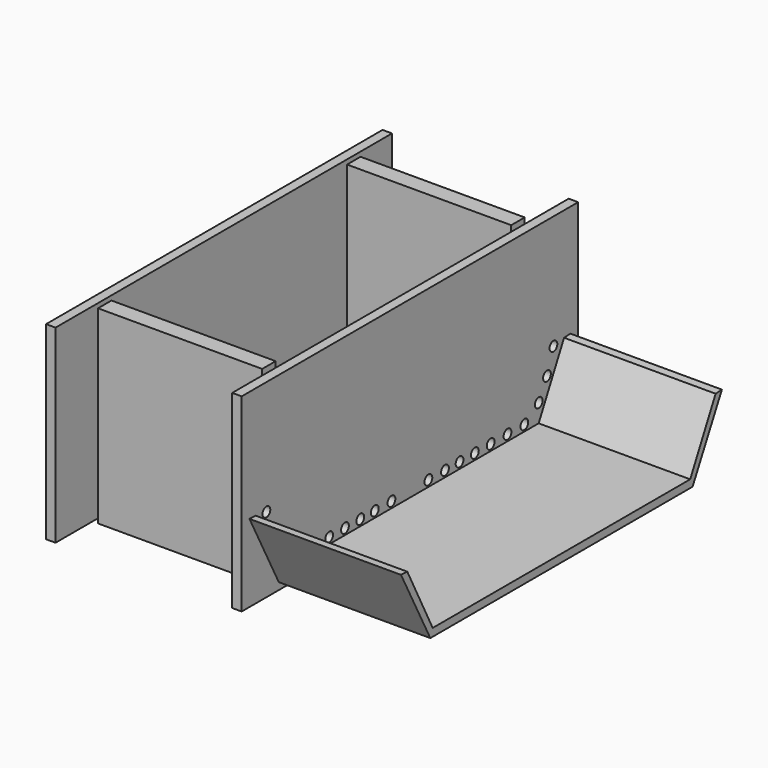
from build123d import *

# Parameters (mm, degrees)
F0_W     = 21.6278625545
F0_H     = 77.5424886208
F1_DEPTH = 10
F0_W_2   = 43.3333408518
F0_H_2   = 4.4457448224
F2_DEPTH = 50
F3_R     = 1.2843906964
F4_DEPTH = 25
F6_DEPTH = 40


with BuildPart() as f1:
    # F0 (on Top) → F1 (new body)
    with BuildSketch(Plane.XY):
        with Locations((10.8139312773, 0)):
            Rectangle(F0_W, F0_H)
        with Locations((-10.8139312773, 0)):
            Rectangle(F0_W, F0_H)
    extrude(amount=F1_DEPTH)


with BuildPart() as f2:
    # F0 (on Top) → F2 (new body)
    with BuildSketch(Plane.XY):
        with Locations((-0.2027006072, 41.0887222738)):
            Rectangle(F0_W_2, F0_H_2)
    extrude(amount=F2_DEPTH)


with BuildPart() as f2b:
    # F0 (on Top) → F2, piece 2 (new body)
    with BuildSketch(Plane.XY):
        Polygon((-23.3169149258, -47.1327573904), (-23.3169149258, 38.7712443104), (-23.3169149258, 47.1327573904), (-23.3169149258, 55.5130317807), (-25.8169149258, 55.5130317807), (-25.8169149258, 47.1327573904), (-25.8169149258, 38.7712443104), (-25.8169149258, -47.1327573904), (-25.8169149258, -55.5130317807), (-23.3169149258, -55.5130317807), align=None)
    extrude(amount=F2_DEPTH)


with BuildPart() as f2c:
    # F0 (on Top) → F2, piece 3 (new body)
    with BuildSketch(Plane.XY):
        Polygon((23.3169149258, 47.1327573904), (23.3169149258, 38.7712443104), (23.3169149258, -47.1327573904), (23.3169149258, -55.5130317807), (25.8169149258, -55.5130317807), (25.8169149258, -47.1327573904), (25.8169149258, 38.7712443104), (25.8169149258, 47.1327573904), (25.8169149258, 55.5130317807), (23.3169149258, 55.5130317807), align=None)
    extrude(amount=F2_DEPTH)

    # F3 (on face) → F4 (cut)
    with BuildSketch(Plane.YZ.offset(25.8169149258)):
        with Locations((-47.3548397422, 19.8441818357)):
            Circle(F3_R)
        with Locations((-45.2270433307, 13.7881413102)):
            Circle(F3_R)
        with Locations((-42.502604425, 8.6867371574)):
            Circle(F3_R)
        with Locations((-37.7573892474, 5.5618393235)):
            Circle(F3_R)
        with Locations((-32.1971963072, 5.5618393235)):
            Circle(F3_R)
        with Locations((-26.6442311032, 5.5618393235)):
            Circle(F3_R)
        with Locations((-21.4299158396, 5.5618393235)):
            Circle(F3_R)
        with Locations((-16.38522475, 5.5618393235)):
            Circle(F3_R)
        with Locations((-11.5741421781, 5.5618393235)):
            Circle(F3_R)
        with Locations((-6.0931830667, 5.5618393235)):
            Circle(F3_R)
        with Locations((6.0931830667, 5.5618393235)):
            Circle(F3_R)
        with Locations((11.5741421781, 5.5618393235)):
            Circle(F3_R)
        with Locations((16.38522475, 5.5618393235)):
            Circle(F3_R)
        with Locations((21.4299158396, 5.5618393235)):
            Circle(F3_R)
        with Locations((26.6442311032, 5.5618393235)):
            Circle(F3_R)
        with Locations((32.1971963072, 5.5618393235)):
            Circle(F3_R)
        with Locations((37.7573892474, 5.5618393235)):
            Circle(F3_R)
        with Locations((42.502604425, 8.6867371574)):
            Circle(F3_R)
        with Locations((45.2270433307, 13.7881413102)):
            Circle(F3_R)
        with Locations((47.3548397422, 19.8441818357)):
            Circle(F3_R)
    extrude(amount=-F4_DEPTH, mode=Mode.SUBTRACT)


with BuildPart() as f2d:
    # F0 (on Top) → F2, piece 4 (new body)
    with BuildSketch(Plane.XY):
        with Locations((-0.2027006072, -41.0887222738)):
            Rectangle(F0_W_2, F0_H_2)
    extrude(amount=F2_DEPTH)


with BuildPart() as f6:
    # F5 (on face) → F6 (new body)
    with BuildSketch(Plane.YZ.offset(25.8169149258)):
        Polygon((-42.4813143909, 3.9014217909), (-50.863917917, 20.3824657947), (-52.9466159642, 20.4923860729), (-43.2693101466, 1.8546198262), (0, 1.8546198262), (0, 3.9014217909), align=None)
        Polygon((42.4813143909, 3.9014217909), (0, 3.9014217909), (0, 1.8546198262), (43.2693101466, 1.8546198262), (52.9466159642, 20.4923860729), (50.863917917, 20.3824657947), align=None)
    extrude(amount=F6_DEPTH)


solid = Compound([f1.part, f2.part, f2b.part, f2c.part, f2d.part, f6.part])
